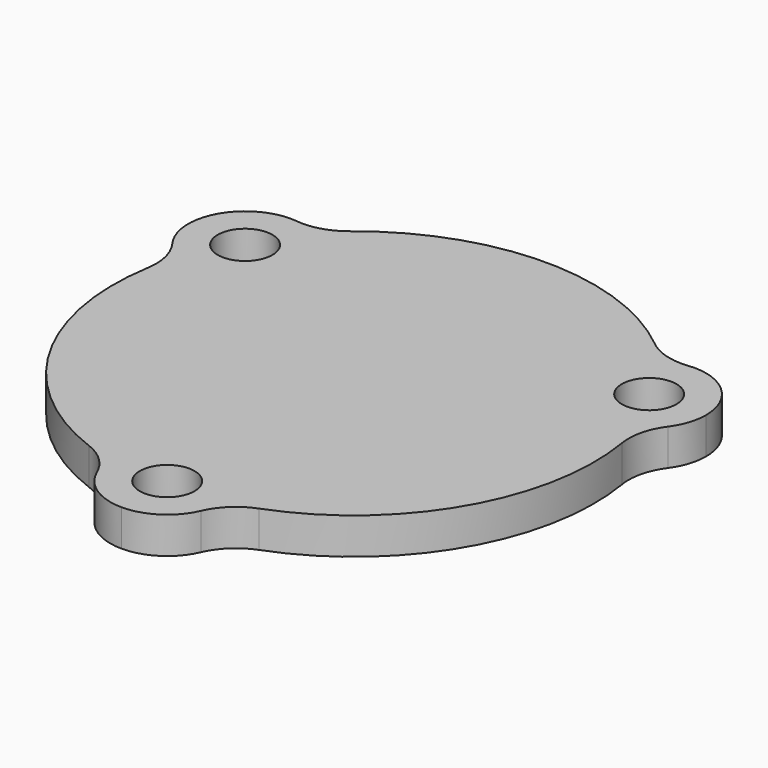
from build123d import *

# Parameters (mm, degrees)
F1_W      = 8.89
F1_H      = 3.175
F3_R      = 2.38125
F4_DEPTH  = 3.176
F7_DEPTH  = 3.176
F8_R      = 5.08
F9_R      = 27.6252152017
F10_DEPTH = 17.4535782288
F11_R     = 14.5350936127
F12_DEPTH = 3.175


# Not quite as in the source:
# - a fillet or chamfer that OpenCascade refuses, or shapes differently, is made with other operations: its cross-section is extruded or revolved along the edge and cut away or added


with BuildPart() as f2:
    # F1 (on Front) → F2 (revolve)
    with BuildSketch(Plane.XZ):
        with BuildLine():
            ThreePointArc((13.208, -11.9177163316), (13.0652297207, -14.7887805254), (12.3057501177, -17.5612494052))
            Line((12.3057501177, -17.5612494052), (16.383, -17.5612494052))
            Line((16.383, -17.5612494052), (16.383, 0))
            Line((16.383, 0), (16.383, 3.175))
            Line((16.383, 3.175), (13.208, 3.175))
            Line((13.208, 3.175), (13.208, -11.9177163316))
        make_face()
        with Locations((20.828, 1.5875)):
            Rectangle(F1_W, F1_H)
    revolve(axis=Axis((0, 0, -9.4681101426), (0, 0, 1)))

    # F3 (on face) → F4 (cut, through all)
    with BuildSketch(Plane(origin=(0, 0, 0), x_dir=(1, 0, 0), z_dir=(0, 0, -1))):
        with BuildLine():
            ThreePointArc((0, 17.93875), (1.6837980227, 18.6362019773), (2.38125, 20.32))
            ThreePointArc((2.38125, 20.32), (-1.6837980227, 22.0037980227), (0, 17.93875))
        make_face()
        with Locations((-17.5976362049, -10.16)):
            Circle(F3_R)
        with Locations((17.5976362049, -10.16)):
            Circle(F3_R)
    extrude(amount=-F4_DEPTH, mode=Mode.SUBTRACT)

    # F5: fillet of radius 5.08 on 1 edges, made by hand

    # F5_s1 → F5_t2 (revolve, cut)
    with BuildSketch(Plane.XZ):
        with BuildLine():
            ThreePointArc((11.303, -17.5612494052), (14.8951024484, -16.0733518536), (16.383, -12.4812494052))
            Line((16.383, -12.4812494052), (16.383, -17.5612494052))
            Line((16.383, -17.5612494052), (11.303, -17.5612494052))
        make_face()
    revolve(axis=Axis((0, 0, -17.5612494052), (0, 0, 1)), mode=Mode.SUBTRACT)

    # F6 (on face) → F7 (cut, through all)
    with BuildSketch(Plane(origin=(0, 0, 0), x_dir=(1, 0, 0), z_dir=(0, 0, -1))):
        with BuildLine():
            ThreePointArc((-4.952964542, 20.3387415379), (-3.495667473, 23.8289197652), (0, 25.273))
            ThreePointArc((0, 25.273), (-21.8870601005, 12.6364998776), (-21.8870598885, -12.6365002448))
            ThreePointArc((-21.8870598885, -12.6365002448), (-22.3842836342, -8.8871231844), (-20.0903491238, -5.8799776515))
            ThreePointArc((-20.0903491238, -5.8799776515), (-18.1286292594, 10.4665689829), (-4.952964542, 20.3387415379))
        make_face()
        with BuildLine():
            ThreePointArc((0, 25.273), (3.495667473, 23.8289197652), (4.952964542, 20.3387415379))
            ThreePointArc((4.952964542, 20.3387415379), (18.1286292594, 10.4665689829), (20.0903491238, -5.8799776515))
            ThreePointArc((20.0903491238, -5.8799776515), (21.8917377458, -7.6916197707), (22.5506362049, -10.16))
            ThreePointArc((22.5506362049, -10.16), (22.3818668231, -11.4419307281), (21.8870600322, -12.6364999959))
            ThreePointArc((21.8870600322, -12.6364999959), (24.4118434084, -6.5411337246), (25.273, 0))
            ThreePointArc((25.273, 0), (17.8707096809, 17.8707096809), (0, 25.273))
        make_face()
        with BuildLine():
            ThreePointArc((-15.1373845818, -14.4587638864), (-18.8886159884, -14.9417967542), (-21.8870598885, -12.6365002448))
            ThreePointArc((-21.8870598885, -12.6365002448), (1.437e-07, -25.273), (21.8870600322, -12.6364999959))
            ThreePointArc((21.8870600322, -12.6364999959), (18.8886161272, -14.9417967167), (15.1373845818, -14.4587638864))
            ThreePointArc((15.1373845818, -14.4587638864), (0, -20.9331379659), (-15.1373845818, -14.4587638864))
        make_face()
    extrude(amount=-F7_DEPTH, mode=Mode.SUBTRACT)

    # F8
    f8_edges = [f2.edges().sort_by_distance(p)[0] for p in [
        (-15.137385, 14.458764, 1.5875),
        (15.137385, 14.458764, 1.5875),
        (20.090349, 5.879978, 1.5875),
        (4.952965, -20.338742, 1.5875),
        (-4.952965, -20.338742, 1.5875),
        (-20.090349, 5.879978, 1.5875),
    ]]
    fillet(f8_edges, radius=F8_R)

    # F9 (on Top) → F10 (cut, through all)
    with BuildSketch(Plane.XY):
        Circle(F9_R)
    extrude(amount=-F10_DEPTH, mode=Mode.SUBTRACT)

    # F11 (on face) → F12 (join)
    with BuildSketch(Plane(origin=(0, 0, 0), x_dir=(1, 0, 0), z_dir=(0, 0, -1))):
        Circle(F11_R)
    extrude(amount=-F12_DEPTH)


solid = f2.part
